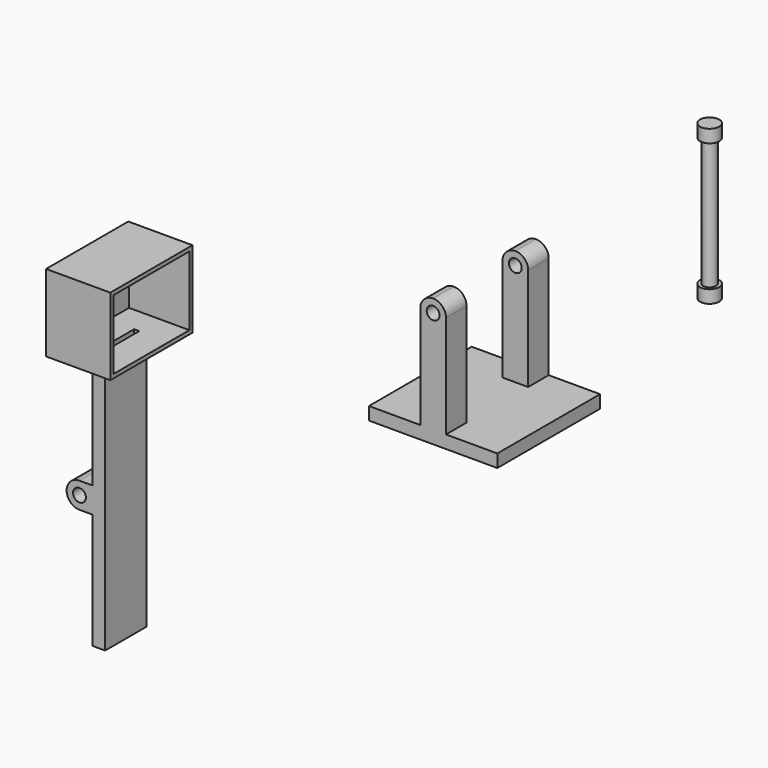
from build123d import *

# Parameters (mm, degrees)
F0_W      = 127
F0_H      = 127
F1_DEPTH  = 12.7
F2_W      = 25.4
F2_H      = 25.4
F3_DEPTH  = 114.3
F4_R      = 12.7
F5_R      = 12.69999
F6_R      = 12.69999
F7_R      = 6.35
F8_DEPTH  = 153.416
F0_R      = 6.35
F9_DEPTH  = 127
F10_R     = 9.525
F11_DEPTH = 12.7
F12_R     = 9.525
F13_DEPTH = 12.7
F0_W_2    = 12.7
F0_H_2    = 50.8
F14_DEPTH = 254
F15_W     = 63.5
F15_H     = 101.6
F15_W_2   = 12.7
F15_H_2   = 50.8
F16_DEPTH = 76.2
F17_T     = -3.81
F18_W     = 50.8
F18_H     = 25.4
F19_DEPTH = 25.4
F20_R     = 12.69999
F21_R     = 6.35
F22_DEPTH = 80.01


# Not quite as in the source:
# - a fillet or chamfer is up to 0.001 mm smaller than in the source, because OpenCascade refuses the exact size


with BuildPart() as f1:
    # F0 (on Top) → F1 (new body)
    with BuildSketch(Plane.XY):
        with Locations((1.2050811201, 8.5559213668)):
            Rectangle(F0_W, F0_H)
    extrude(amount=F1_DEPTH)

    # F2 (on face) → F3 (join)
    with BuildSketch(Plane.XY.offset(12.7)):
        with Locations((1.2050811201, -42.2440786332)):
            Rectangle(F2_W, F2_H)
        with Locations((1.2050811201, 59.3559213668)):
            Rectangle(F2_W, F2_H)
    extrude(amount=F3_DEPTH)

    # F4
    f4_edges = [f1.edges().sort_by_distance(p)[0] for p in [
        (13.905081, -42.244079, 127),
    ]]
    fillet(f4_edges, radius=F4_R)

    # F5 (radius 12.7 in the source; OpenCascade refuses exactly that, so slightly less here)
    f5_edges = [f1.edges().sort_by_distance(p)[0] for p in [
        (-11.494919, -42.244079, 127),
    ]]
    fillet(f5_edges, radius=F5_R)

    # F6 (radius 12.7 in the source; OpenCascade refuses exactly that, so slightly less here)
    f6_edges = [f1.edges().sort_by_distance(p)[0] for p in [
        (-11.494919, 59.355921, 127),
        (13.905081, 59.355921, 127),
    ]]
    fillet(f6_edges, radius=F6_R)

    # F7 (on face) → F8 (cut)
    with BuildSketch(Plane.XZ.offset(54.9440786332)):
        with Locations((1.2050811201, 114.3)):
            Circle(F7_R)
    extrude(amount=-F8_DEPTH, mode=Mode.SUBTRACT)


with BuildPart() as f9:
    # F0 (on Top) → F9 (new body)
    with BuildSketch(Plane.XY):
        with Locations((0, 288.3246541023)):
            Circle(F0_R)
    extrude(amount=F9_DEPTH)

    # F10 (on face) → F11 (join)
    with BuildSketch(Plane.XY.offset(127)):
        with Locations((0, 288.3246541023)):
            Circle(F10_R)
    extrude(amount=F11_DEPTH)

    # F12 (on face) → F13 (join)
    with BuildSketch(Plane(origin=(0, 0, 0), x_dir=(1, 0, 0), z_dir=(0, 0, -1))):
        with Locations((0, -288.3246541023)):
            Circle(F12_R)
    extrude(amount=F13_DEPTH)


with BuildPart() as f14:
    # F0 (on Top) → F14 (new body)
    with BuildSketch(Plane.XY):
        with Locations((12.5742597342, -457.1122058392)):
            Rectangle(F0_W_2, F0_H_2)
    extrude(amount=F14_DEPTH)

    # F15 (on face) → F16 (join)
    with BuildSketch(Plane.XY.offset(254)):
        with Locations((12.5742597342, -457.1122058392)):
            Rectangle(F15_W, F15_H)
        with Locations((12.5742597342, -457.1122058392)):
            Rectangle(F15_W_2, F15_H_2, mode=Mode.SUBTRACT)
        with Locations((12.5742597342, -457.1122058392)):
            Rectangle(F15_W_2, F15_H_2)
    extrude(amount=F16_DEPTH)

    # F17
    f17_openings = [f14.faces().sort_by_distance(p)[0] for p in [
        (44.32426, -457.112206, 292.1),
    ]]
    offset(amount=F17_T, openings=f17_openings, kind=Kind.INTERSECTION)

    # F18 (on face) → F19 (join)
    with BuildSketch(Plane(origin=(6.2242597342, 0, 0), x_dir=(0, -1, 0), z_dir=(-1, 0, 0))):
        with Locations((457.1122058392, 127)):
            Rectangle(F18_W, F18_H)
    extrude(amount=F19_DEPTH)

    # F20 (radius 12.7 in the source; OpenCascade refuses exactly that, so slightly less here)
    f20_edges = [f14.edges().sort_by_distance(p)[0] for p in [
        (-19.17574, -457.112206, 114.3),
        (-19.17574, -457.112206, 139.7),
    ]]
    fillet(f20_edges, radius=F20_R)

    # F21 (on face) → F22 (cut)
    with BuildSketch(Plane.XZ.offset(482.5122058392)):
        with Locations((-6.4757402658, 127)):
            Circle(F21_R)
    extrude(amount=-F22_DEPTH, mode=Mode.SUBTRACT)


solid = Compound([f1.part, f9.part, f14.part])
